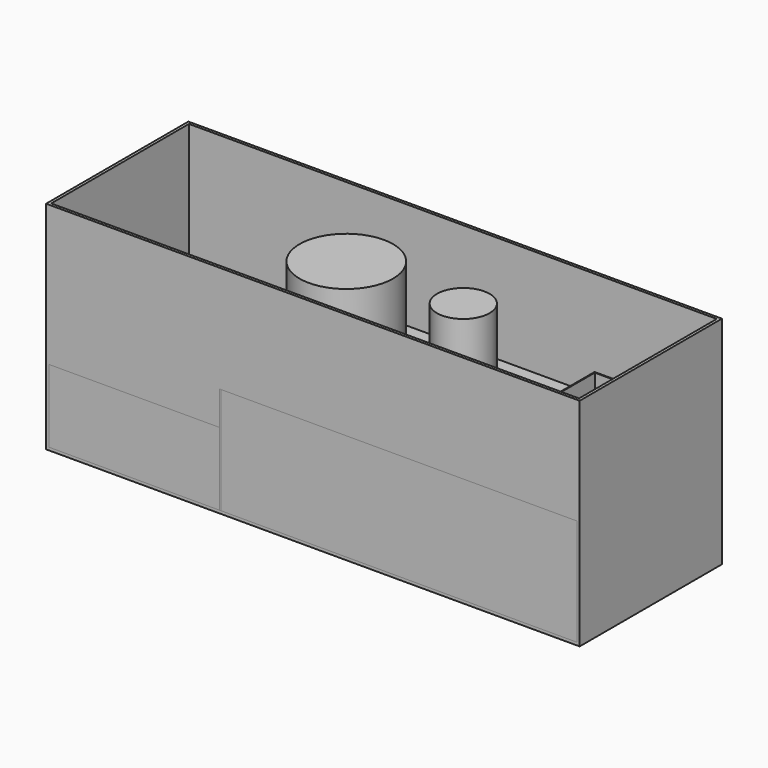
from build123d import *

# Parameters (mm, degrees)
F0_W           = 1500
F0_H           = 500
F0_W_2         = 1484
F0_H_2         = 484
F1_DEPTH       = 8
F2_DEPTH       = 600
F4_W           = 5
F4_H           = 300
F5_DEPTH       = 492
F7_DEPTH       = 200
F7_DEPTH_BACK  = 200
F8_T           = -2.5
F10_R          = 131.4761602714
F11_DEPTH      = 500
F10_R_2        = 73.8496876532
F12_W          = 193.4688985348
F12_H          = 106.2804311514
F13_DEPTH      = 100
F14_R          = 20
F15_DEPTH      = 243
F16_W          = 1000
F16_H          = 300
F17_DEPTH      = 250
F17_DEPTH_BACK = 242
F16_W_2        = 479
F16_H_2        = 204.8108279705
F18_W          = 608.7850779295
F18_H          = 355.7835072279
F19_DEPTH      = 100
F20_DEPTH      = 242
F20_DEPTH_BACK = 242


with BuildPart() as f1:
    # F0 (on Top) → F1 (new body)
    with BuildSketch(Plane.XY):
        Rectangle(F0_W, F0_H)
        Rectangle(F0_W_2, F0_H_2, mode=Mode.SUBTRACT)
        Rectangle(F0_W_2, F0_H_2)
    extrude(amount=-F1_DEPTH)


with BuildPart() as f2:
    # F0 (on Top) → F2 (new body)
    with BuildSketch(Plane.XY):
        Rectangle(F0_W, F0_H)
        Rectangle(F0_W_2, F0_H_2, mode=Mode.SUBTRACT)
    extrude(amount=F2_DEPTH)


with BuildPart() as f1_1:
    add(f1.part)

    # F3: union F2
    add(f2.part)


with BuildPart() as f5:
    # F4 (on face) → F5 (new body, through all)
    with BuildSketch(Plane.XZ.offset(250)):
        with Locations((-260.5, 150)):
            Rectangle(F4_W, F4_H)
    extrude(amount=-F5_DEPTH)


with BuildPart() as f7:
    # F6 (on Front) → F7 (new body, two sides)
    with BuildSketch(Plane.XZ) as f7_sk:
        Polygon((432, 235), (472, 235), (702, 235), (742, 235), (742, 385), (432, 385), align=None)
    extrude(amount=-F7_DEPTH)
    extrude(f7_sk.sketch, amount=F7_DEPTH_BACK)

    # F8
    f8_openings = [f7.faces().sort_by_distance(p)[0] for p in [
        (587, 0, 385),
    ]]
    offset(amount=F8_T, openings=f8_openings)

    # F14 (on face) → F15 (join, through all)
    with BuildSketch(Plane(origin=(0, 0, 235), x_dir=(1, 0, 0), z_dir=(0, 0, -1))):
        with Locations((482, 150)):
            Circle(F14_R)
        with Locations((692, 150)):
            Circle(F14_R)
        with Locations((692, -150)):
            Circle(F14_R)
        with Locations((482, -150)):
            Circle(F14_R)
    extrude(amount=F15_DEPTH)


with BuildPart() as f11:
    # F10 (on offset) → F11 (new body)
    with BuildSketch(Plane.XY.offset(100)):
        with Locations((-64.0354678035, -52.4545870721)):
            Circle(F10_R)
    extrude(amount=F11_DEPTH)


with BuildPart() as f11b:
    # F10 (on offset) → F11, piece 2 (new body)
    with BuildSketch(Plane.XY.offset(100)):
        with Locations((261.5916728973, -48.3672171831)):
            Circle(F10_R_2)
    extrude(amount=F11_DEPTH)


with BuildPart() as f13:
    # F12 (on face) → F13 (new body)
    with BuildSketch(Plane.XY):
        with Locations((-576.319232583, 116.8514415622)):
            Rectangle(F12_W, F12_H)
    extrude(amount=F13_DEPTH)


with BuildPart() as f17:
    # F16 (on Front) → F17 (new body, two sides)
    with BuildSketch(Plane.XZ) as f17_sk:
        with Locations((242, 150)):
            Rectangle(F16_W, F16_H)
    extrude(amount=F17_DEPTH)
    extrude(f17_sk.sketch, amount=-F17_DEPTH_BACK)


with BuildPart() as f17b:
    # F16 (on Front) → F17, piece 2 (new body, two sides)
    with BuildSketch(Plane.XZ) as f17_2_sk:
        with Locations((-502.5, 102.4054139853)):
            Rectangle(F16_W_2, F16_H_2)
    extrude(amount=F17_DEPTH)
    extrude(f17_2_sk.sketch, amount=-F17_DEPTH_BACK)

    # F16 (on Front) → F20 (join, two sides)
    with BuildSketch(Plane.XZ) as f20_sk:
        with Locations((-502.5, 102.4054139853)):
            Rectangle(F16_W_2, F16_H_2)
    extrude(amount=-F20_DEPTH)
    extrude(f20_sk.sketch, amount=F20_DEPTH_BACK)


with BuildPart() as f19:
    # F18 (on offset) → F19 (new body, through all)
    with BuildSketch(Plane.XY.offset(100)):
        with Locations((81.0395553708, -36.5666374564)):
            Rectangle(F18_W, F18_H)
    extrude(amount=-F19_DEPTH)


solid = Compound([f1_1.part, f5.part, f7.part, f11.part, f11b.part, f13.part, f17.part, f17b.part, f19.part])
